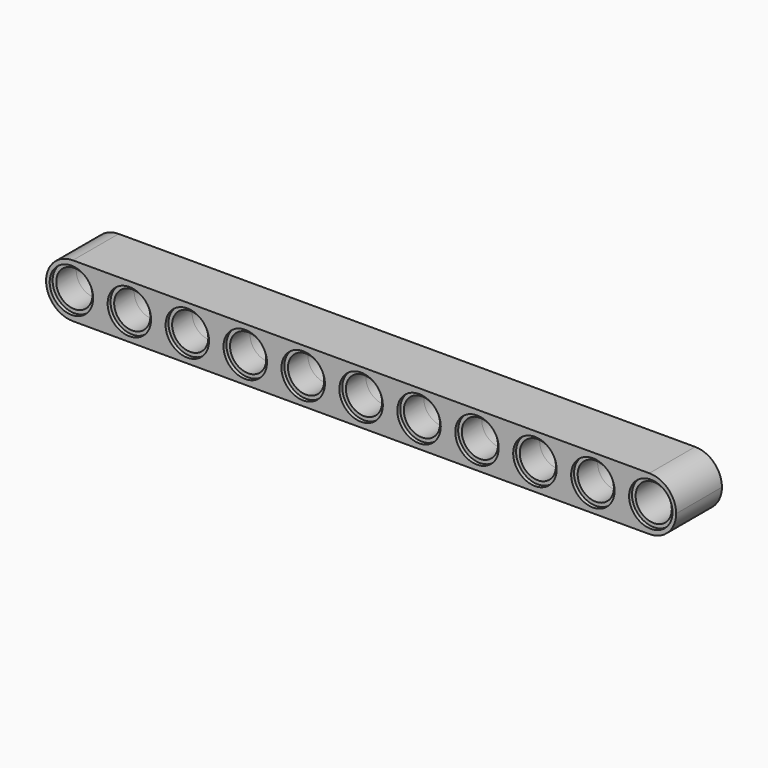
from build123d import *

# Parameters (mm, degrees)
F0_R     = 3
F1_DEPTH = 3.95
F0_R_2   = 2.499
F2_DEPTH = 3.45
F3_R     = 3.69999
F4_R     = 3.69999


# Not quite as in the source:
# - a fillet or chamfer is up to 0.001 mm smaller than in the source, because OpenCascade refuses the exact size


with BuildPart() as f1:
    # F0 (on Front) → F1 (new body, symmetric)
    with BuildSketch(Plane.XZ):
        Polygon((-43.5, 0), (0, 0), (43.5, 0), (43.5, 7.4), (-43.5, 7.4), align=None)
        with Locations((-40, 3.7)):
            Circle(F0_R, mode=Mode.SUBTRACT)
        with Locations((-32, 3.7)):
            Circle(F0_R, mode=Mode.SUBTRACT)
        with Locations((-24, 3.7)):
            Circle(F0_R, mode=Mode.SUBTRACT)
        with Locations((-16, 3.7)):
            Circle(F0_R, mode=Mode.SUBTRACT)
        with Locations((-8, 3.7)):
            Circle(F0_R, mode=Mode.SUBTRACT)
        with Locations((0, 3.7)):
            Circle(F0_R, mode=Mode.SUBTRACT)
        with Locations((8, 3.7)):
            Circle(F0_R, mode=Mode.SUBTRACT)
        with Locations((16, 3.7)):
            Circle(F0_R, mode=Mode.SUBTRACT)
        with Locations((24, 3.7)):
            Circle(F0_R, mode=Mode.SUBTRACT)
        with Locations((32, 3.7)):
            Circle(F0_R, mode=Mode.SUBTRACT)
        with Locations((40, 3.7)):
            Circle(F0_R, mode=Mode.SUBTRACT)
    extrude(amount=F1_DEPTH, both=True)

    # F0 (on Front) → F2 (join, symmetric)
    with BuildSketch(Plane.XZ):
        with Locations((-40, 3.7)):
            Circle(F0_R)
        with Locations((-40, 3.7)):
            Circle(F0_R_2, mode=Mode.SUBTRACT)
        with Locations((-32, 3.7)):
            Circle(F0_R)
        with Locations((-32, 3.7)):
            Circle(F0_R_2, mode=Mode.SUBTRACT)
        with Locations((-24, 3.7)):
            Circle(F0_R)
        with Locations((-24, 3.7)):
            Circle(F0_R_2, mode=Mode.SUBTRACT)
        with Locations((-16, 3.7)):
            Circle(F0_R)
        with Locations((-16, 3.7)):
            Circle(F0_R_2, mode=Mode.SUBTRACT)
        with Locations((-8, 3.7)):
            Circle(F0_R)
        with Locations((-8, 3.7)):
            Circle(F0_R_2, mode=Mode.SUBTRACT)
        with Locations((0, 3.7)):
            Circle(F0_R)
        with Locations((0, 3.7)):
            Circle(F0_R_2, mode=Mode.SUBTRACT)
        with Locations((8, 3.7)):
            Circle(F0_R)
        with Locations((8, 3.7)):
            Circle(F0_R_2, mode=Mode.SUBTRACT)
        with Locations((16, 3.7)):
            Circle(F0_R)
        with Locations((16, 3.7)):
            Circle(F0_R_2, mode=Mode.SUBTRACT)
        with Locations((24, 3.7)):
            Circle(F0_R)
        with Locations((24, 3.7)):
            Circle(F0_R_2, mode=Mode.SUBTRACT)
        with Locations((32, 3.7)):
            Circle(F0_R)
        with Locations((32, 3.7)):
            Circle(F0_R_2, mode=Mode.SUBTRACT)
        with Locations((40, 3.7)):
            Circle(F0_R)
        with Locations((40, 3.7)):
            Circle(F0_R_2, mode=Mode.SUBTRACT)
    extrude(amount=F2_DEPTH, both=True)

    # F3 (radius 3.7 in the source; OpenCascade refuses exactly that, so slightly less here)
    f3_edges = [f1.edges().sort_by_distance(p)[0] for p in [
        (-43.5, 0, 7.4),
        (-43.5, 0, 0),
    ]]
    fillet(f3_edges, radius=F3_R)

    # F4 (radius 3.7 in the source; OpenCascade refuses exactly that, so slightly less here)
    f4_edges = [f1.edges().sort_by_distance(p)[0] for p in [
        (43.5, 0, 7.4),
        (43.5, 0, 0),
    ]]
    fillet(f4_edges, radius=F4_R)


solid = f1.part
